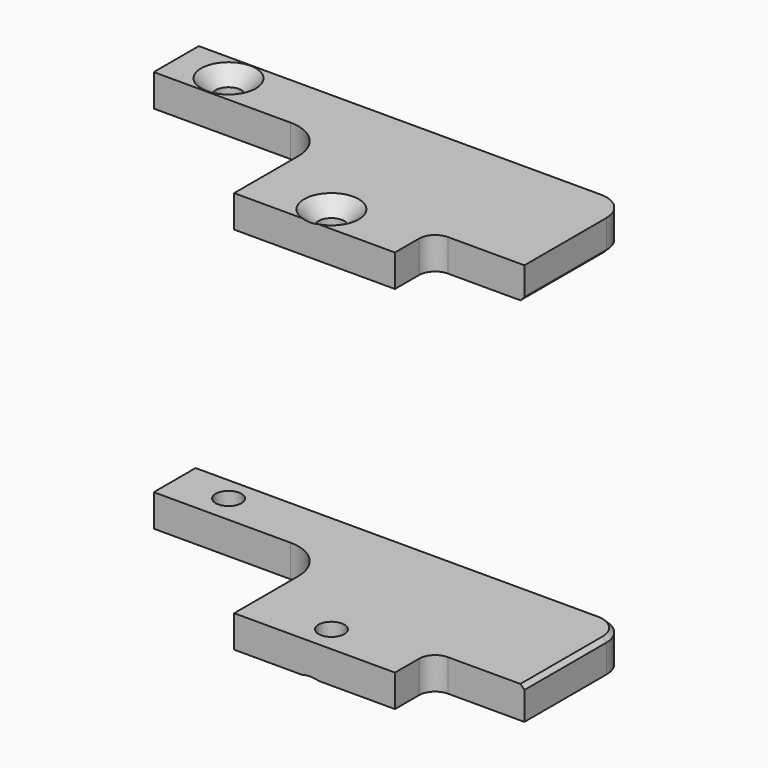
from build123d import *

# Parameters (mm, degrees)
F0_W      = 42
F0_H      = 22
F1_DEPTH  = 4
F2_W      = 29
F2_H      = 16.25
F3_DEPTH  = 4
F4_R      = 3.5
F5_R      = 2
F6_R      = 1.6
F7_DEPTH  = 25
F8_W      = 22
F8_H      = 15
F9_DEPTH  = 25
F10_R     = 5
F11_R     = 1.6
F12_DEPTH = 25
F15_SIZE  = 0.5


# Not quite as in the source:
# - a fillet or chamfer that OpenCascade refuses, or shapes differently, is made with other operations: its cross-section is extruded or revolved along the edge and cut away or added


with BuildPart() as f1:
    # F0 (on Top) → F1 (new body)
    with BuildSketch(Plane.XY):
        with Locations((21, -11)):
            Rectangle(F0_W, F0_H)
    extrude(amount=F1_DEPTH)

    # F2 (on Top) → F3 (join)
    with BuildSketch(Plane.XY):
        with Locations((39, -8.125)):
            Rectangle(F2_W, F2_H)
    extrude(amount=F3_DEPTH)

    # F4
    f4_edges = [f1.edges().sort_by_distance(p)[0] for p in [
        (53.5, 0, 2),
    ]]
    fillet(f4_edges, radius=F4_R)

    # F5
    f5_edges = [f1.edges().sort_by_distance(p)[0] for p in [
        (42, -16.25, 2),
    ]]
    fillet(f5_edges, radius=F5_R)

    # F6 (on face) → F7 (cut)
    with BuildSketch(Plane.XY.offset(4)):
        with Locations((6.5, -3.5)):
            Circle(F6_R)
    extrude(amount=-F7_DEPTH, mode=Mode.SUBTRACT)

    # F8 (on face) → F9 (cut)
    with BuildSketch(Plane.XY.offset(4)):
        with Locations((11, -14.5)):
            Rectangle(F8_W, F8_H)
    extrude(amount=-F9_DEPTH, mode=Mode.SUBTRACT)

    # F10
    f10_edges = [f1.edges().sort_by_distance(p)[0] for p in [
        (22, -7, 2),
    ]]
    fillet(f10_edges, radius=F10_R)

    # F11 (on face) → F12 (cut)
    with BuildSketch(Plane.XY.offset(4)):
        with Locations((31.5, -18.75)):
            Circle(F11_R)
    extrude(amount=-F12_DEPTH, mode=Mode.SUBTRACT)

    # F14: chamfer of 1.8 on 2 edges, made by hand

    # F14_s1 → F14_t2 (revolve, cut)
    with BuildSketch(Plane.XZ.offset(18.75)):
        Polygon((34.9, 0), (33.1, 1.8), (33.1, 0), align=None)
    revolve(axis=Axis((31.5, -18.75, 0), (0, 0, 1)), mode=Mode.SUBTRACT)

    # F14_s3 → F14_t4 (revolve, cut)
    with BuildSketch(Plane.XZ.offset(3.5)):
        Polygon((9.9, 0), (8.1, 1.8), (8.1, 0), align=None)
    revolve(axis=Axis((6.5, -3.5, 0), (0, 0, 1)), mode=Mode.SUBTRACT)

    # F15
    f15_edges = [f1.edges().sort_by_distance(p)[0] for p in [
        (53.5, -9.875, 4),
        (52.474874, -1.025126, 4),
        (25, 0, 4),
    ]]
    chamfer(f15_edges, length=F15_SIZE)


with BuildPart() as f16_1:
    # F16: instance of F1
    add(f1.part.mirror(Plane.XY.offset(25)))


solid = Compound([f1.part, f16_1.part])
